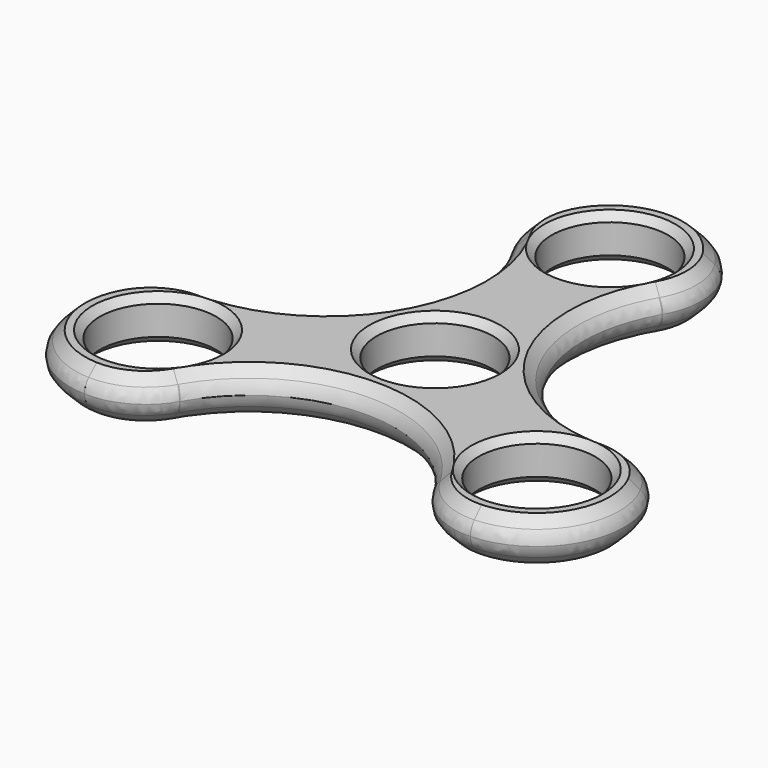
from build123d import *

# Parameters (mm, degrees)
F0_R     = 8
F1_DEPTH = 6
F2_SIZE  = 2
F3_R     = 2.399


# Not quite as in the source:
# - a fillet or chamfer that OpenCascade refuses, or shapes differently, is made with other operations: its cross-section is extruded or revolved along the edge and cut away or added
# - a fillet or chamfer is up to 0.001 mm smaller than in the source, because OpenCascade refuses the exact size


with BuildPart() as f1:
    # F0 (on Top) → F1 (new body)
    with BuildSketch(Plane.XY):
        with BuildLine():
            ThreePointArc((17.3752396583, -21.9506129232), (21.2176246931, -25.7460968589), (26.473346357, -26.9898857694))
            ThreePointArc((26.473346357, -26.9898857694), (36.3730669589, -21), (36.6105999, -9.4316475837))
            ThreePointArc((36.6105999, -9.4316475837), (32.9055862747, -5.5019535627), (27.6974082493, -4.0720924793))
            ThreePointArc((27.6974082493, -4.0720924793), (10.266913183, 5.9276050899), (10.322168591, 26.0227054025))
            ThreePointArc((10.322168591, 26.0227054025), (11.6879615816, 31.2480504217), (10.137253543, 36.4215333531))
            ThreePointArc((10.137253543, 36.4215333531), (0, 42), (-10.137253543, 36.4215333531))
            ThreePointArc((-10.137253543, 36.4215333531), (-11.6879615816, 31.2480504217), (-10.322168591, 26.0227054025))
            ThreePointArc((-10.322168591, 26.0227054025), (-10.266913183, 5.9276050899), (-27.6974082493, -4.0720924793))
            ThreePointArc((-27.6974082493, -4.0720924793), (-32.9055862747, -5.5019535627), (-36.6105999, -9.4316475837))
            ThreePointArc((-36.6105999, -9.4316475837), (-36.3730669589, -21), (-26.473346357, -26.9898857694))
            ThreePointArc((-26.473346357, -26.9898857694), (-21.2176246931, -25.7460968589), (-17.3752396583, -21.9506129232))
            ThreePointArc((-17.3752396583, -21.9506129232), (0, -11.8552101799), (17.3752396583, -21.9506129232))
        make_face()
        with Locations((-25.9807621135, -15)):
            Circle(F0_R, mode=Mode.SUBTRACT)
        with Locations((25.9807621135, -15)):
            Circle(F0_R, mode=Mode.SUBTRACT)
        Circle(F0_R, mode=Mode.SUBTRACT)
        with Locations((0, 30)):
            Circle(F0_R, mode=Mode.SUBTRACT)
    extrude(amount=F1_DEPTH)

    # F2
    f2_edges = [f1.edges().sort_by_distance(p)[0] for p in [
        (-10.266913, 5.927605, 6),
        (-11.687962, 31.24805, 6),
        (0, 42, 6),
        (11.687962, 31.24805, 6),
        (10.266913, 5.927605, 6),
        (32.905586, -5.501954, 6),
        (36.373067, -21, 6),
        (21.217625, -25.746097, 6),
        (0, -11.85521, 6),
        (-21.217625, -25.746097, 6),
        (-36.373067, -21, 6),
        (-32.905586, -5.501954, 6),
        (-21.217625, -25.746097, 0),
        (-36.373067, -21, 0),
        (-32.905586, -5.501954, 0),
        (-10.266913, 5.927605, 0),
        (-11.687962, 31.24805, 0),
        (0, -11.85521, 0),
        (21.217625, -25.746097, 0),
        (36.373067, -21, 0),
        (32.905586, -5.501954, 0),
        (10.266913, 5.927605, 0),
        (11.687962, 31.24805, 0),
        (0, 42, 0),
        (27.697408, -4.072092, 3),
        (10.322169, 26.022705, 3),
    ]]
    chamfer(f2_edges, length=F2_SIZE)

    # F3 (radius 2.4 in the source; OpenCascade refuses exactly that, so slightly less here)
    f3_edges = [f1.edges().sort_by_distance(p)[0] for p in [
        (27.697408, -4.072092, 3),
        (10.266913, 5.927605, 2),
        (10.266913, 5.927605, 4),
        (10.322169, 26.022705, 3),
        (36.6106, -9.431648, 3),
        (32.905586, -5.501954, 2),
        (32.905586, -5.501954, 4),
        (26.473346, -26.989886, 3),
        (36.373067, -21, 2),
        (36.373067, -21, 4),
        (17.37524, -21.950613, 3),
        (21.217625, -25.746097, 2),
        (21.217625, -25.746097, 4),
        (-17.37524, -21.950613, 3),
        (0, -11.85521, 2),
        (0, -11.85521, 4),
        (-26.473346, -26.989886, 3),
        (-21.217625, -25.746097, 2),
        (-21.217625, -25.746097, 4),
        (-36.6106, -9.431648, 3),
        (-36.373067, -21, 2),
        (-36.373067, -21, 4),
        (-27.697408, -4.072092, 3),
        (-32.905586, -5.501954, 2),
        (-32.905586, -5.501954, 4),
        (-10.322169, 26.022705, 3),
        (-10.266913, 5.927605, 2),
        (-10.266913, 5.927605, 4),
        (-10.137254, 36.421533, 3),
        (-11.687962, 31.24805, 2),
        (-11.687962, 31.24805, 4),
        (10.137254, 36.421533, 3),
        (0, 42, 2),
        (0, 42, 4),
        (11.687962, 31.24805, 2),
        (11.687962, 31.24805, 4),
    ]]
    fillet(f3_edges, radius=F3_R)

    # F4: chamfer of 1 on 12 edges, made by hand

    # F4_s1 → F4_t2 (revolve, cut)
    with BuildSketch(Plane.XZ.offset(-30)):
        Polygon((9, 0), (8, 1), (8, 0), align=None)
    revolve(axis=Axis((0, 30, 0), (0, 0, 1)), mode=Mode.SUBTRACT)

    # F4_s3 → F4_t4 (revolve, cut)
    with BuildSketch(Plane.XZ.offset(-30)):
        Polygon((9, 6), (8, 5), (8, 6), align=None)
    revolve(axis=Axis((0, 30, 6), (0, 0, 1)), mode=Mode.SUBTRACT)

    # F4_s5 → F4_t6 (revolve, cut)
    with BuildSketch(Plane.XZ.offset(15)):
        Polygon((34.9807621135, 0), (33.9807621135, 1), (33.9807621135, 0), align=None)
    revolve(axis=Axis((25.9807621135, -15, 0), (0, 0, 1)), mode=Mode.SUBTRACT)

    # F4_s7 → F4_t8 (revolve, cut)
    with BuildSketch(Plane.XZ.offset(15)):
        Polygon((34.9807621135, 6), (33.9807621135, 5), (33.9807621135, 6), align=None)
    revolve(axis=Axis((25.9807621135, -15, 6), (0, 0, 1)), mode=Mode.SUBTRACT)

    # F4_s9 → F4_t10 (revolve, cut)
    with BuildSketch(Plane.XZ):
        Polygon((9, 0), (8, 1), (8, 0), align=None)
    revolve(axis=Axis((0, 0, 0), (0, 0, 1)), mode=Mode.SUBTRACT)

    # F4_s11 → F4_t12 (revolve, cut)
    with BuildSketch(Plane.XZ):
        Polygon((9, 6), (8, 5), (8, 6), align=None)
    revolve(axis=Axis((0, 0, 6), (0, 0, 1)), mode=Mode.SUBTRACT)

    # F4_s13 → F4_t14 (revolve, cut)
    with BuildSketch(Plane.XZ.offset(15)):
        Polygon((-16.9807621135, 0), (-17.9807621135, 1), (-17.9807621135, 0), align=None)
    revolve(axis=Axis((-25.9807621135, -15, 0), (0, 0, 1)), mode=Mode.SUBTRACT)

    # F4_s15 → F4_t16 (revolve, cut)
    with BuildSketch(Plane.XZ.offset(15)):
        Polygon((-16.9807621135, 6), (-17.9807621135, 5), (-17.9807621135, 6), align=None)
    revolve(axis=Axis((-25.9807621135, -15, 6), (0, 0, 1)), mode=Mode.SUBTRACT)


solid = f1.part
